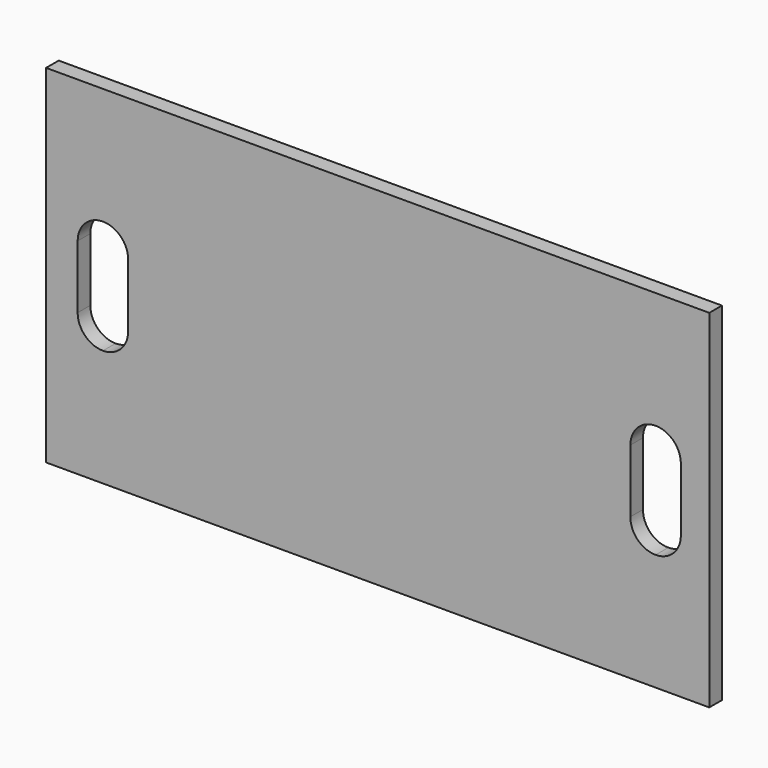
from build123d import *

# Parameters (mm, degrees)
F0_W     = 210
F0_H     = 110
F0_W_2   = 16
F0_H_2   = 36
F1_DEPTH = 5
F2_R     = 7.99999


# Not quite as in the source:
# - a fillet or chamfer is up to 0.001 mm smaller than in the source, because OpenCascade refuses the exact size
# - a feature names something its author has since deleted; it is built from what else it names


with BuildPart() as f1:
    # F0 (on Front) → F1 (new body)
    with BuildSketch(Plane.XZ):
        Rectangle(F0_W, F0_H)
        with Locations((-87, 0)):
            Rectangle(F0_W_2, F0_H_2, mode=Mode.SUBTRACT)
        with Locations((88, 0)):
            Rectangle(F0_W_2, F0_H_2, mode=Mode.SUBTRACT)
    extrude(amount=F1_DEPTH)

    # F2 (radius 8 in the source; OpenCascade refuses exactly that, so slightly less here)
    f2_edges = [f1.edges().sort_by_distance(p)[0] for p in [
        (-95, -2.5, 18),
        (-79, -2.5, 18),
        (-95, -2.5, -18),
        (-79, -2.5, -18),
        (80, -2.5, 18),
        (96, -2.5, 18),
        (96, -2.5, -18),
        (80, -2.5, -18),
    ]]
    fillet(f2_edges, radius=F2_R)


solid = f1.part
